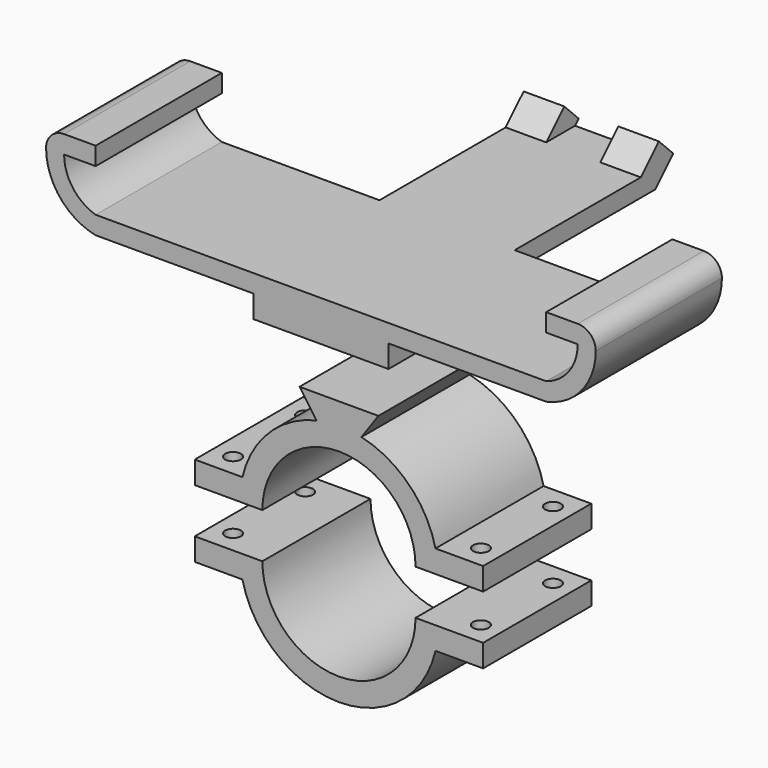
from build123d import *

# Parameters (mm, degrees)
F3_DEPTH      = 30
F4_DEPTH      = 5
F6_DEPTH      = 15
F6_DEPTH_BACK = 15
F7_DEPTH      = 6
F8_DEPTH      = 30
F9_DEPTH      = 30
F10_R         = 1.75
F11_DEPTH     = 50


# Not quite as in the source:
# - a feature names something its author has since deleted; it is built from what else it names


with BuildPart() as f3:
    # F2 (on offset) → F3 (new body)
    with BuildSketch(Plane.XZ.offset(30)):
        with BuildLine():
            Line((50, 49), (-50, 49))
            ThreePointArc((-50, 49), (-55.0610018108, 52.5997881394), (-57, 58.5))
            Line((-57, 58.5), (-50, 58.5))
            Line((-50, 58.5), (-50, 62.5))
            Line((-50, 62.5), (-57, 62.5))
            ThreePointArc((-57, 62.5), (-59.8284271247, 61.3284271247), (-61, 58.5))
            ThreePointArc((-61, 58.5), (-57.9018186072, 49.7929626164), (-50, 45))
            Line((-50, 45), (-15, 45))
            Line((-15, 45), (-15, 40))
            Line((-15, 40), (-5.748962309, 40))
            Line((-5.748962309, 40), (-9.25, 45))
            Line((-9.25, 45), (9.25, 45))
            Line((9.25, 45), (5.748962309, 40))
            Line((5.748962309, 40), (15, 40))
            Line((15, 40), (15, 45))
            Line((15, 45), (50, 45))
            ThreePointArc((50, 45), (57.9018186072, 49.7929626164), (61, 58.5))
            ThreePointArc((61, 58.5), (59.8284271247, 61.3284271247), (57, 62.5))
            Line((57, 62.5), (50, 62.5))
            Line((50, 62.5), (50, 58.5))
            Line((50, 58.5), (57, 58.5))
            ThreePointArc((57, 58.5), (55.0610018108, 52.5997881394), (50, 49))
        make_face()
    extrude(amount=-F3_DEPTH)

    # F2 (on offset) → F4 (join)
    with BuildSketch(Plane.XZ.offset(30)):
        with BuildLine():
            Line((50, 49), (-50, 49))
            ThreePointArc((-50, 49), (-55.0610018108, 52.5997881394), (-57, 58.5))
            Line((-57, 58.5), (-50, 58.5))
            Line((-50, 58.5), (-50, 62.5))
            Line((-50, 62.5), (-57, 62.5))
            ThreePointArc((-57, 62.5), (-59.8284271247, 61.3284271247), (-61, 58.5))
            ThreePointArc((-61, 58.5), (-57.9018186072, 49.7929626164), (-50, 45))
            Line((-50, 45), (-15, 45))
            Line((-15, 45), (-15, 40))
            Line((-15, 40), (-5.748962309, 40))
            Line((-5.748962309, 40), (-9.25, 45))
            Line((-9.25, 45), (9.25, 45))
            Line((9.25, 45), (5.748962309, 40))
            Line((5.748962309, 40), (15, 40))
            Line((15, 40), (15, 45))
            Line((15, 45), (50, 45))
            ThreePointArc((50, 45), (57.9018186072, 49.7929626164), (61, 58.5))
            ThreePointArc((61, 58.5), (59.8284271247, 61.3284271247), (57, 62.5))
            Line((57, 62.5), (50, 62.5))
            Line((50, 62.5), (50, 58.5))
            Line((50, 58.5), (57, 58.5))
            ThreePointArc((57, 58.5), (55.0610018108, 52.5997881394), (50, 49))
        make_face()
        Polygon((-9.25, 45), (-5.748962309, 40), (5.748962309, 40), (9.25, 45), align=None)
    extrude(amount=F4_DEPTH)

    # F5 (on Right) → F6 (join, two sides)
    with BuildSketch(Plane.YZ) as f6_sk:
        Polygon((35, 49), (0, 49), (0, 45), (39, 45), (43, 49), align=None)
        Polygon((40, 54), (35, 49), (43, 49), (44, 50), align=None)
    extrude(amount=F6_DEPTH)
    extrude(f6_sk.sketch, amount=-F6_DEPTH_BACK)

    # F5 (on Right) → F7 (cut, symmetric)
    with BuildSketch(Plane.YZ):
        Polygon((40, 54), (35, 49), (43, 49), (44, 50), align=None)
    extrude(amount=F7_DEPTH, both=True, mode=Mode.SUBTRACT)


with BuildPart() as f8:
    # F0 (on Front) → F8 (new body)
    with BuildSketch(Plane.XZ):
        with BuildLine():
            Line((-32, 0), (-22, 0))
            ThreePointArc((-22, 0), (-21.8555974099, 2.516517804), (-21.4242852856, 5))
            Line((-21.4242852856, 5), (-32, 5))
            Line((-32, 5), (-32, 0))
        make_face()
        with BuildLine():
            Line((-22, 0), (-17, 0))
            Line((-17, 0), (-17, 5))
            Line((-17, 5), (-21.4242852856, 5))
            ThreePointArc((-21.4242852856, 5), (-21.8555974099, 2.516517804), (-22, 0))
        make_face()
        with BuildLine():
            ThreePointArc((-17, 0), (0, 17), (17, 0))
            Line((17, 0), (17, 5))
            Line((17, 5), (21.4242852856, 5))
            ThreePointArc((21.4242852856, 5), (15.5563491861, 15.5563491861), (5, 21.4242852856))
            ThreePointArc((5, 21.4242852856), (0, 22), (-5, 21.4242852856))
            ThreePointArc((-5, 21.4242852856), (-15.5563491861, 15.5563491861), (-21.4242852856, 5))
            Line((-21.4242852856, 5), (-17, 5))
            Line((-17, 5), (-17, 0))
        make_face()
        with BuildLine():
            Line((17, 5), (17, 0))
            Line((17, 0), (22, 0))
            ThreePointArc((22, 0), (21.8555974099, 2.516517804), (21.4242852856, 5))
            Line((21.4242852856, 5), (17, 5))
        make_face()
        with BuildLine():
            ThreePointArc((21.4242852856, 5), (21.8555974099, 2.516517804), (22, 0))
            Line((22, 0), (32, 0))
            Line((32, 0), (32, 5))
            Line((32, 5), (21.4242852856, 5))
        make_face()
        with BuildLine():
            ThreePointArc((-5, 21.4242852856), (0, 22), (5, 21.4242852856))
            Line((5, 21.4242852856), (8.75, 26.7798403109))
            Line((8.75, 26.7798403109), (-8.75, 26.7798403109))
            Line((-8.75, 26.7798403109), (-5, 21.4242852856))
        make_face()
    extrude(amount=F8_DEPTH)


with BuildPart() as f9:
    # F0 (on Front) → F9 (new body)
    with BuildSketch(Plane.XZ):
        with BuildLine():
            ThreePointArc((-21.4242852856, -15), (-21.8555974099, -12.516517804), (-22, -10))
            Line((-22, -10), (-32, -10))
            Line((-32, -10), (-32, -15))
            Line((-32, -15), (-21.4242852856, -15))
        make_face()
        with BuildLine():
            Line((-17, -15), (-17, -10))
            Line((-17, -10), (-22, -10))
            ThreePointArc((-22, -10), (-21.8555974099, -12.516517804), (-21.4242852856, -15))
            Line((-21.4242852856, -15), (-17, -15))
        make_face()
        with BuildLine():
            ThreePointArc((17, -10), (0, -27), (-17, -10))
            Line((-17, -10), (-17, -15))
            Line((-17, -15), (-21.4242852856, -15))
            ThreePointArc((-21.4242852856, -15), (0, -32), (21.4242852856, -15))
            Line((21.4242852856, -15), (17, -15))
            Line((17, -15), (17, -10))
        make_face()
        with BuildLine():
            Line((22, -10), (17, -10))
            Line((17, -10), (17, -15))
            Line((17, -15), (21.4242852856, -15))
            ThreePointArc((21.4242852856, -15), (21.8555974099, -12.516517804), (22, -10))
        make_face()
        with BuildLine():
            Line((32, -10), (22, -10))
            ThreePointArc((22, -10), (21.8555974099, -12.516517804), (21.4242852856, -15))
            Line((21.4242852856, -15), (32, -15))
            Line((32, -15), (32, -10))
        make_face()
    extrude(amount=F9_DEPTH)


with BuildPart() as f11_tool:
    # F10 (on face) → F11 (new body)
    with BuildSketch(Plane.XY.offset(5)):
        with Locations((-27.5, -25)):
            Circle(F10_R)
        with Locations((-27.5, -5)):
            Circle(F10_R)
        with Locations((27.5, -5)):
            Circle(F10_R)
        with Locations((27.5, -25)):
            Circle(F10_R)
    extrude(amount=-F11_DEPTH)


with BuildPart() as f8_1:
    add(f8.part)

    # F11: cut by f11_tool
    add(f11_tool.part, mode=Mode.SUBTRACT)


with BuildPart() as f9_1:
    add(f9.part)

    # F11: cut by f11_tool
    add(f11_tool.part, mode=Mode.SUBTRACT)


solid = Compound([f3.part, f8_1.part, f9_1.part])
